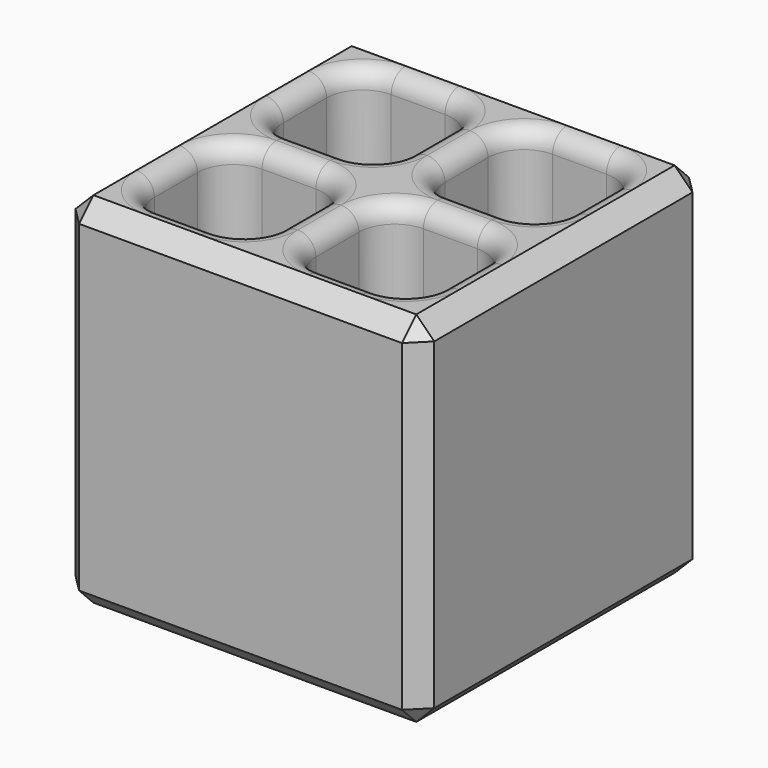
from build123d import *

# Parameters (mm, degrees)
F0_W     = 100
F0_H     = 100
F1_DEPTH = 100
F2_T     = -10
F3_W     = 35
F3_H     = 10
F3_W_2   = 10
F3_H_2   = 35
F4_DEPTH = 90
F5_SIZE  = 5
F6_R     = 10
F7_R     = 4.99999


# Not quite as in the source:
# - a fillet or chamfer is up to 0.001 mm smaller than in the source, because OpenCascade refuses the exact size


with BuildPart() as f1:
    # F0 (on Top) → F1 (new body)
    with BuildSketch(Plane.XY):
        Rectangle(F0_W, F0_H)
    extrude(amount=F1_DEPTH)

    # F2
    f2_openings = [f1.faces().sort_by_distance(p)[0] for p in [
        (0, 0, 100),
    ]]
    offset(amount=F2_T, openings=f2_openings)

    # F3 (on face) → F4 (join, through all)
    with BuildSketch(Plane.XY.offset(100)):
        with Locations((-22.5, 0)):
            Rectangle(F3_W, F3_H)
        Rectangle(F3_W_2, F3_H)
        with Locations((0, -22.5)):
            Rectangle(F3_W_2, F3_H_2)
        with Locations((0, 22.5)):
            Rectangle(F3_W_2, F3_H_2)
        with Locations((22.5, 0)):
            Rectangle(F3_W, F3_H)
    extrude(amount=-F4_DEPTH)

    # F5
    f5_edges = [f1.edges().sort_by_distance(p)[0] for p in [
        (50, 0, 100),
        (0, -50, 100),
        (0, 50, 100),
        (-50, 0, 100),
        (50, -50, 50),
        (50, 0, 0),
        (0, -50, 0),
        (-50, -50, 50),
        (-50, 0, 0),
        (-50, 50, 50),
        (0, 50, 0),
        (50, 50, 50),
    ]]
    chamfer(f5_edges, length=F5_SIZE)

    # F6
    f6_edges = [f1.edges().sort_by_distance(p)[0] for p in [
        (-40, -40, 55),
        (-40, -22.5, 10),
        (-40, -5, 55),
        (-22.5, -5, 10),
        (-5, -22.5, 10),
        (-22.5, -40, 10),
        (-5, -5, 55),
        (-5, -40, 55),
        (-40, 5, 55),
        (-40, 22.5, 10),
        (-22.5, 5, 10),
        (-40, 40, 55),
        (-22.5, 40, 10),
        (-5, 22.5, 10),
        (-5, 5, 55),
        (-5, 40, 55),
        (5, -22.5, 10),
        (5, 22.5, 10),
        (22.5, 40, 10),
        (5, 40, 55),
        (5, 5, 55),
        (22.5, 5, 10),
        (40, 40, 55),
        (40, 22.5, 10),
        (40, 5, 55),
        (5, -5, 55),
        (22.5, -5, 10),
        (5, -40, 55),
        (22.5, -40, 10),
        (40, -22.5, 10),
        (40, -5, 55),
        (40, -40, 55),
    ]]
    fillet(f6_edges, radius=F6_R)

    # F7 (radius 5 in the source; OpenCascade refuses exactly that, so slightly less here)
    f7_edges = [f1.edges().sort_by_distance(p)[0] for p in [
        (-40, -22.5, 100),
        (-40, 22.5, 100),
        (5, 22.5, 100),
        (5, -22.5, 100),
    ]]
    fillet(f7_edges, radius=F7_R)


solid = f1.part
